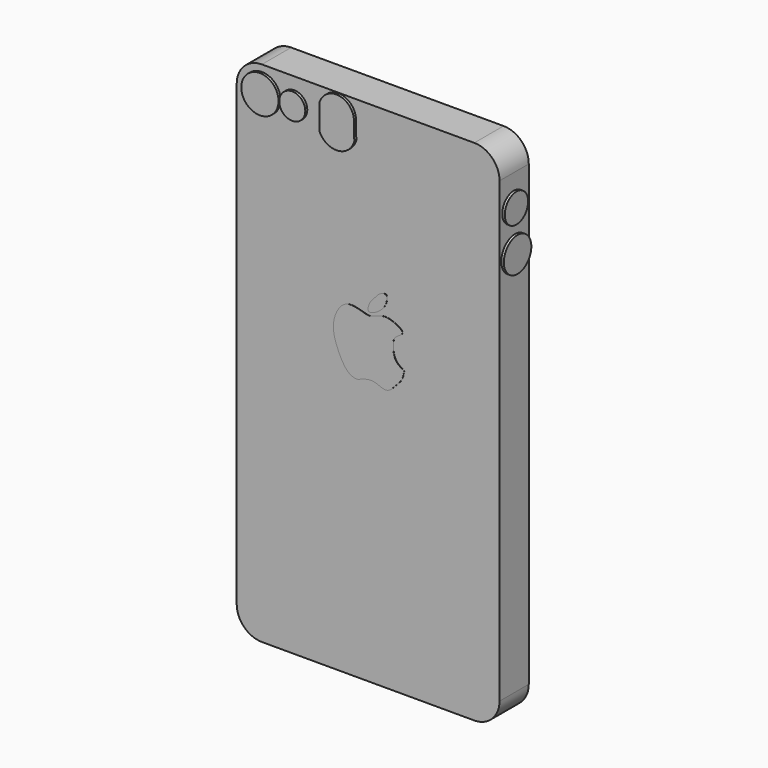
from build123d import *

# Parameters (mm, degrees)
F0_W      = 52.9562598094
F0_H      = 102.458845824
F1_DEPTH  = 7.366
F2_R      = 5.08
F4_R      = 2.6590711811
F4_W      = 9.4277970493
F4_H      = 3.8080494851
F4_R_2    = 2.2218501958
F5_DEPTH  = 25.4
F3_R      = 3.9983268575
F6_DEPTH  = 0.3175
F8_DEPTH  = 7.112
F9_R      = 3.7522124086
F10_DEPTH = 0.508
F9_R_2    = 2.6194678396
F11_DEPTH = 0.508
F13_DEPTH = 7.366
F14_R     = 2.927204105
F14_W     = 29.4005014002
F14_H     = 3.302000463
F14_R_2   = 1.0239087259
F15_DEPTH = 0.508
F18_DEPTH = 0.0508
F19_R     = 2.9350553776
F20_DEPTH = 0.508


# Not quite as in the source:
# - a feature of the source that left no trace in its solid (it failed there, or was rolled back) is left out


with BuildPart() as f1:
    # F0 (on Front) → F1 (new body)
    with BuildSketch(Plane.XZ):
        with Locations((-19.2829859443, -1.1512245983)):
            Rectangle(F0_W, F0_H)
    extrude(amount=F1_DEPTH)

    # F2
    f2_edges = [f1.edges().sort_by_distance(p)[0] for p in [
        (-45.761116, -3.683, 50.078198),
        (7.195144, -3.683, 50.078198),
        (7.195144, -3.683, -52.380648),
        (-45.761116, -3.683, -52.380648),
    ]]
    fillet(f2_edges, radius=F2_R)

    # F4 (on face) → F5 (cut)
    with BuildSketch(Plane(origin=(0, 0, -52.3806475103), x_dir=(1, 0, 0), z_dir=(0, 0, -1))):
        with Locations((-2.3175266106, 3.70877143)):
            Circle(F4_R)
        with Locations((-20.9451001137, 4.031334538)):
            Rectangle(F4_W, F4_H)
        with Locations((-35.6035269797, 3.8380967453)):
            Circle(F4_R_2)
    extrude(amount=-F5_DEPTH, mode=Mode.SUBTRACT)

    # F3 (on face) → F6 (cut)
    with BuildSketch(Plane(origin=(0, 0, 0), x_dir=(-1, 0, 0), z_dir=(0, 1, 0))):
        with Locations((19.2829859443, -46.756785363)):
            Circle(F3_R)
    extrude(amount=-F6_DEPTH, mode=Mode.SUBTRACT)

    # F7 (on face) → F8 (cut)
    with BuildSketch(Plane(origin=(0, 0, 0), x_dir=(-1, 0, 0), z_dir=(0, 1, 0))):
        Polygon((39.8780032992, 40.6373552978), (-3.3019997645, 40.6373552978), (-3.8099999074, -39.6266467869), (39.8780032992, -39.6266467869), align=None)
    extrude(amount=-F8_DEPTH, mode=Mode.SUBTRACT)

    # F9 (on face) → F10 (join)
    with BuildSketch(Plane.XZ.offset(7.366)):
        with Locations((-40.681115849, 44.9981983137)):
            Circle(F9_R)
    extrude(amount=F10_DEPTH)

    # F9 (on face) → F11 (join)
    with BuildSketch(Plane.XZ.offset(7.366)):
        with Locations((-40.681115849, 44.9981983137)):
            Circle(F9_R)
        with BuildLine():
            Line((-21.6612099299, 42.8335605604), (-21.757948526, 46.8708315703))
            ThreePointArc((-21.757948526, 46.8708315703), (-24.9186836694, 49.9411794414), (-28.6305304617, 47.56642133))
            Line((-28.6305304617, 47.56642133), (-28.6305304617, 42.2230027616))
            ThreePointArc((-28.6305304617, 42.2230027616), (-24.9319153156, 40.0860556465), (-21.6612099299, 42.8335605604))
        make_face()
        with Locations((-34.1592803597, 44.9981983137)):
            Circle(F9_R_2)
    extrude(amount=F11_DEPTH)

    # F14 (on face) → F15 (cut)
    with BuildSketch(Plane(origin=(0, 0, 0), x_dir=(-1, 0, 0), z_dir=(0, 1, 0))):
        with Locations((2.3924480192, 45.2824570239)):
            Circle(F14_R)
        with Locations((20.7121986896, 44.5204563439)):
            Rectangle(F14_W, F14_H)
        with Locations((19.727949053, 47.5049614906)):
            Circle(F14_R_2)
    extrude(amount=-F15_DEPTH, mode=Mode.SUBTRACT)

    # F17 (on face) → F18 (join)
    with BuildSketch(Plane.XZ.offset(7.366)):
        with BuildLine():
            add(Edge.make_bspline(
                [(-12.313099578, 11.7068113759), (-12.3182719745, 11.2693172346), (-14.0471777892, 10.6426821522), (-14.1694497269, 9.1976154433), (-14.1923588981, 7.8253429333), (-13.757045673, 6.2502584285), (-12.732998031, 5.4901288014), (-11.7868601393, 4.9184492153), (-12.0625993678, 4.9249552084), (-12.1356791253, 3.442670809), (-13.4938891698, 2.1372915784), (-14.6469691571, 0.7161487492), (-15.8059393346, 0.355170558), (-16.8810715776, 0.7668398235), (-18.1810906095, 1.2782789872), (-19.4231192534, 1.1799743607), (-20.6034478055, 0.8441669396), (-21.4837195128, 0.3523397632), (-23.1053492827, 0.8727222184), (-24.3238470967, 2.3773718388), (-25.5506684803, 4.8598592274), (-26.5539056297, 8.0644702423), (-25.7467847595, 11.4294737742), (-23.2717151551, 14.0857698999), (-19.2198549823, 12.2943314765), (-18.2008775604, 12.7833222733), (-16.4425818501, 13.4295862797), (-14.8558748752, 13.5055890759), (-12.3067060672, 12.2475904084), (-12.313099578, 11.7068113759)],
                knots=[0, 0, 0, 0, 0.0391492889, 0.0727778694, 0.1067456455, 0.1424756723, 0.1765910088, 0.203123685, 0.2108828285, 0.2430017031, 0.2838259394, 0.3225995677, 0.3526017684, 0.3829884004, 0.4168954172, 0.4489787383, 0.4805794524, 0.5087166076, 0.5441864617, 0.5839082017, 0.6318706413, 0.6843397655, 0.737125556, 0.7879855348, 0.8446273684, 0.8747593402, 0.9123058727, 0.951608233, 1, 1, 1, 1], degree=3))
        make_face()
        with BuildLine():
            add(Edge.make_bspline(
                [(-17.779443413, 16.2513870746), (-17.5596513889, 16.4997277835), (-17.2523909762, 17.0381238074), (-15.2307876048, 17.9329802627), (-15.5028451921, 15.7361114376), (-16.3303567014, 14.6029182381), (-17.5839563283, 13.5203805258), (-19.6950391667, 12.8825060067), (-18.857112639, 15.3017670358), (-18.0476883571, 15.9482999183), (-17.779443413, 16.2513870746)],
                knots=[0, 0, 0, 0, 0.1034730724, 0.2289362231, 0.3537312944, 0.4791233423, 0.6151717915, 0.7370776987, 0.8737163979, 1, 1, 1, 1], degree=3))
        make_face()
    extrude(amount=F18_DEPTH)

    # F19 (on face) → F20 (join)
    with BuildSketch(Plane.YZ.offset(7.1951439604)):
        with Locations((-3.741475055, 38.8537757099)):
            Circle(F19_R)
        with BuildLine():
            Line((0, 30.2196182314), (0, 30.7952016589))
            ThreePointArc((0, 30.7952016589), (-6.9193087342, 30.5074099451), (0, 30.2196182314))
        make_face()
    extrude(amount=F20_DEPTH)


with BuildPart() as f13:
    # F12 (on face) → F13 (new body)
    with BuildSketch(Plane(origin=(0, -7.112, 0), x_dir=(-1, 0, 0), z_dir=(0, 1, 0))):
        Polygon((39.8780032992, -39.6266467869), (39.8780032992, 40.6373552978), (-3.3019997645, 40.6373552978), (-3.8099999074, -39.6266467869), align=None)
    extrude(amount=F13_DEPTH)


solid = Compound([f1.part, f13.part])
